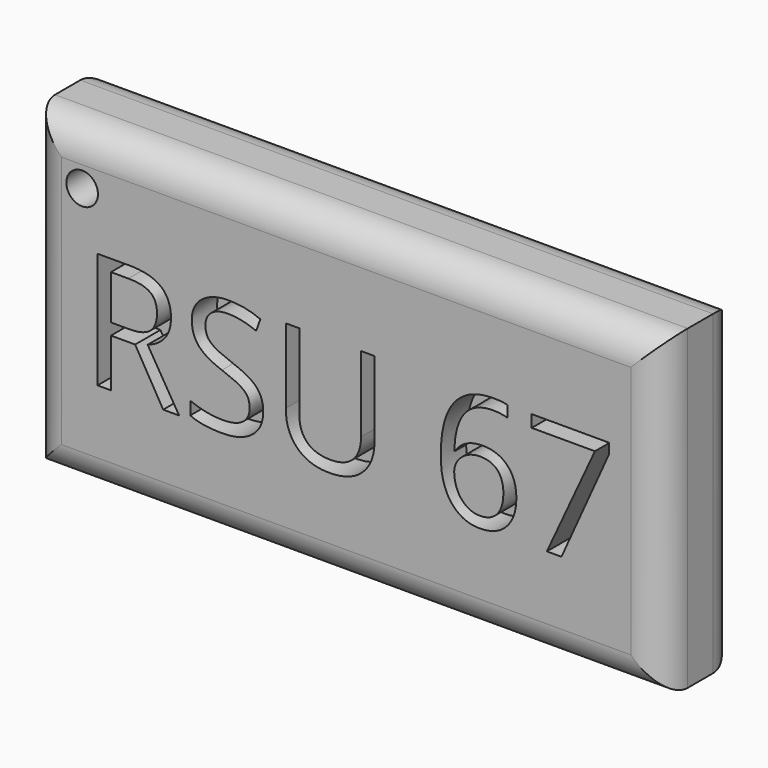
from build123d import *

# Parameters (mm, degrees)
F0_W         = 100
F0_H         = 50
F1_DEPTH     = 15
F2_R         = 5
F3_R         = 2.5
F4_DEPTH     = 15.001
F5_TEXT_SIZE = 25.6615878107
F6_DEPTH     = 5


# Not quite as in the source:
# - Text() gives the source's letters only with a copy of the font that has no kerning and outlines rounded to 1/6400 em; it was checked with that copy


with BuildPart() as f1:
    # F0 (on Front) → F1 (new body)
    with BuildSketch(Plane.XZ):
        Rectangle(F0_W, F0_H)
    extrude(amount=F1_DEPTH)

    # F2
    f2_edges = [f1.edges().sort_by_distance(p)[0] for p in [
        (0, -15, 25),
        (50, -15, 0),
        (0, -15, -25),
        (-50, -15, 0),
        (0, 0, 25),
        (-50, 0, 0),
        (0, 0, -25),
        (50, 0, 0),
    ]]
    fillet(f2_edges, radius=F2_R)

    # F3 (on face) → F4 (cut, through all)
    with BuildSketch(Plane.XZ.offset(15)):
        with Locations((-41.7, 16.7)):
            Circle(F3_R)
    extrude(amount=-F4_DEPTH, mode=Mode.SUBTRACT)

    # F5 (on face) → F6 (cut)
    with BuildSketch(Plane.XZ.offset(15)):
        with Locations((-41.7993939358, -9.9169058815)):
            Text('RSU 67', F5_TEXT_SIZE, font='Open Sans', text_align=(TextAlign.LEFT, TextAlign.BOTTOM))
    extrude(amount=-F6_DEPTH, mode=Mode.SUBTRACT)


solid = f1.part
